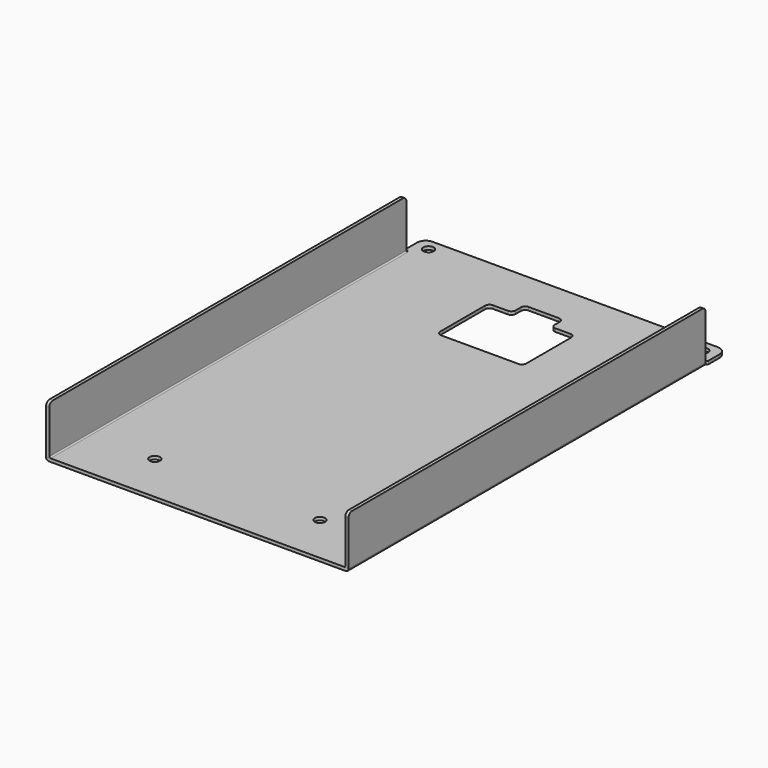
from build123d import *

# Parameters (mm, degrees)
F1_R     = 1.2
F2_DEPTH = 0.744
F3_W     = 0.744
F3_H     = 103
F3_H_2   = 103.0000144269
F4_DEPTH = 12
F5_R     = 1
F6_W     = 0.744
F6_H     = 0.5
F7_DEPTH = 25
F8_R     = 0.3
F9_R     = 0.65
F10_R    = 0.3


# Not quite as in the source:
# - ends of sketch curves that miss each other by under 0.0002 mm in the source are joined


with BuildPart() as f2:
    # F1 (on Top) → F2 (new body)
    with BuildSketch(Plane.XY):
        with BuildLine():
            Line((-39.500012, -54.4999965731), (30.29995, -54.5000015731))
            Line((30.29995, -54.5000015731), (30.29995, 52.5000044269))
            ThreePointArc((30.29995, 52.5000044269), (29.7141635624, 53.9142179893), (28.29995, 54.5000044269))
            Line((28.29995, 54.5000044269), (-37.500012, 54.5000044269))
            ThreePointArc((-37.500012, 54.5000044269), (-38.9142255624, 53.9142179893), (-39.500012, 52.5000044269))
            Line((-39.500012, 52.5000044269), (-39.500012, -54.4999965731))
        make_face()
        with Locations((-23.649861, -42.9501055731)):
            Circle(F1_R, mode=Mode.SUBTRACT)
        with Locations((14.450063, -42.9501055731)):
            Circle(F1_R, mode=Mode.SUBTRACT)
        with Locations((-36.250012, 51.7500052865)):
            Circle(F1_R, mode=Mode.SUBTRACT)
        with BuildLine():
            Line((0.899969, 41.9500044269), (4.34995, 41.9500044269))
            ThreePointArc((4.34995, 41.9500044269), (5.0570567812, 41.6571112081), (5.34995, 40.9500044269))
            Line((5.34995, 40.9500044269), (5.34995, 27.9500044269))
            ThreePointArc((5.34995, 27.9500044269), (5.0570567812, 27.2428976457), (4.34995, 26.9500044269))
            Line((4.34995, 26.9500044269), (-13.55005, 26.9500044269))
            ThreePointArc((-13.55005, 26.9500044269), (-14.2571567812, 27.2428976457), (-14.55005, 27.9500044269))
            Line((-14.55005, 27.9500044269), (-14.55005, 40.9500044269))
            ThreePointArc((-14.55005, 40.9500044269), (-14.2571567812, 41.6571112081), (-13.55005, 41.9500044269))
            Line((-13.55005, 41.9500044269), (-10.100031, 41.9500044269))
            ThreePointArc((-10.100031, 41.9500044269), (-9.3929242188, 42.2428976457), (-9.100031, 42.9500044269))
            Line((-9.100031, 42.9500044269), (-9.100031, 44.4500044269))
            ThreePointArc((-9.100031, 44.4500044269), (-8.8071377812, 45.1571112081), (-8.100031, 45.4500044269))
            Line((-8.100031, 45.4500044269), (-4.600031, 45.4500044269))
            Line((-4.600031, 45.4500044269), (-1.100031, 45.4500044269))
            ThreePointArc((-1.100031, 45.4500044269), (-0.3929242188, 45.1571112081), (-0.100031, 44.4500044269))
            Line((-0.100031, 44.4500044269), (-0.100031, 42.9500044269))
            ThreePointArc((-0.100031, 42.9500044269), (0.1928622188, 42.2428976457), (0.899969, 41.9500044269))
        make_face(mode=Mode.SUBTRACT)
        with Locations((27.04995, 51.750023553)):
            Circle(F1_R, mode=Mode.SUBTRACT)
    extrude(amount=F2_DEPTH)

    # F3 (on face) → F4 (join)
    with BuildSketch(Plane(origin=(0, 0, 0), x_dir=(1, 0, 0), z_dir=(0, 0, -1))):
        with Locations((29.92795, 2.9999821461)):
            Rectangle(F3_W, F3_H)
        with Locations((-39.128012, 2.9999893596)):
            Rectangle(F3_W, F3_H_2)
    extrude(amount=-F4_DEPTH)

    # F5
    f5_edges = [f2.edges().sort_by_distance(p)[0] for p in [
        (29.92795, -54.499982, 12),
        (29.92795, 48.500018, 12),
        (-39.128012, 48.500018, 12),
        (-39.128012, -54.499997, 12),
    ]]
    fillet(f5_edges, radius=F5_R)

    # F6 (on face) → F7 (cut)
    with BuildSketch(Plane.XY.offset(0.744)):
        with Locations((-39.128012, 48.7500178539)):
            Rectangle(F6_W, F6_H)
        with Locations((29.92795, 48.7500178539)):
            Rectangle(F6_W, F6_H)
    extrude(amount=-F7_DEPTH, mode=Mode.SUBTRACT)

    # F8
    f8_edges = [f2.edges().sort_by_distance(p)[0] for p in [
        (30.29995, 49.000018, 0.372),
        (29.55595, 49.000018, 0.372),
        (-39.500012, 49.000018, 0.372),
        (-38.756012, 49.000018, 0.372),
    ]]
    fillet(f8_edges, radius=F8_R)

    # F9
    f9_edges = [f2.edges().sort_by_distance(p)[0] for p in [
        (-39.500012, -2.999989, 0),
        (30.29995, -2.999992, 0),
    ]]
    fillet(f9_edges, radius=F9_R)

    # F10
    f10_edges = [f2.edges().sort_by_distance(p)[0] for p in [
        (-38.756012, -2.999989, 0.744),
        (29.55595, -2.999982, 0.744),
    ]]
    fillet(f10_edges, radius=F10_R)


solid = f2.part
